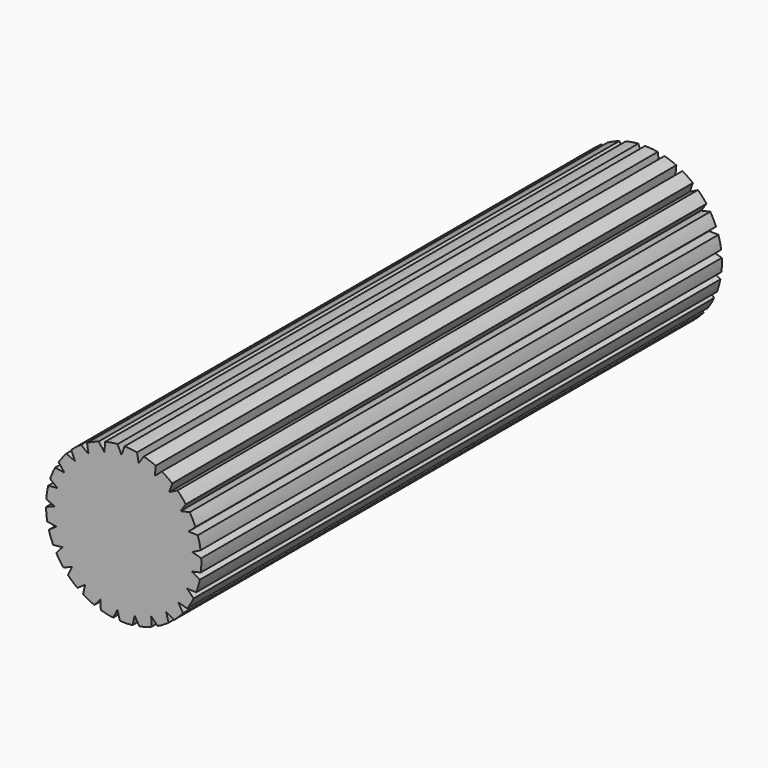
from build123d import *

# Parameters (mm, degrees)
F0_R            = 47.752
F1_DEPTH        = 400.304
F3_DEPTH        = 400.305
F3_COPIES_COUNT = 25


# Not quite as in the source:
# - a pattern or mirror of a feature is missing from the dataset's text; its kind, count and spacing are read off the source's solid


with BuildPart() as f1:
    # F0 (on Front) → F1 (new body)
    with BuildSketch(Plane.XZ):
        Circle(F0_R)
    extrude(amount=F1_DEPTH)

    # F2 (on face) → F3 (cut, through all)
    with BuildSketch(Plane(origin=(0, 0, 0), x_dir=(-1, 0, 0), z_dir=(0, 1, 0))):
        Polygon((-9.1665348659, 41.3941448169), (-6.7116842624, 56.5903173732), (-17.8075077925, 54.133200462), align=None)
    f3 = extrude(amount=-F3_DEPTH, mode=Mode.SUBTRACT)

    # F3_copies: F3 ×25 about axis
    f3_copies_axis = Axis((0, 0, 0), (0, 1, 0))
    for i in range(1, F3_COPIES_COUNT):
        add(f3.rotate(f3_copies_axis, i * 360 / F3_COPIES_COUNT), mode=Mode.SUBTRACT)


solid = f1.part
